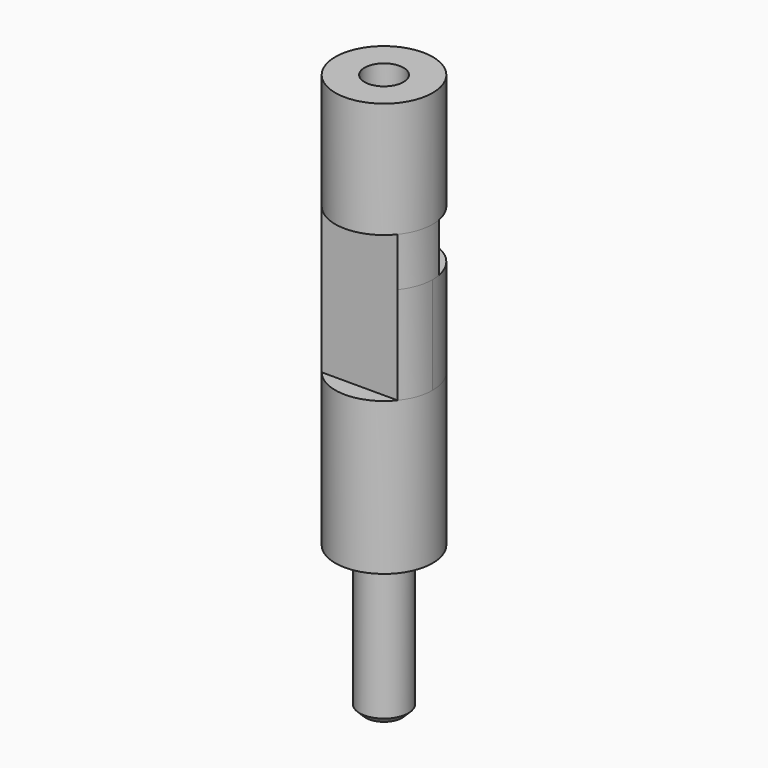
from build123d import *
from build123d import SkipClean  # not in build123d's __all__

# Parameters (mm, degrees)
F2_SIZE   = 0.5
F4_DEPTH  = 8
F6_DEPTH  = 4
F7_R      = 4
F8_DEPTH  = 9.5
F10_D     = 3.2
F10_DEPTH = 14
F10_TIP   = 0.9613769904
F11_R     = 1.6
F12_DEPTH = 2.53


# Not quite as in the source:
# - after a boolean that leaves OpenCascade's solid faulty, fix() repairs it


with BuildPart() as f1:
    # F0 (on Front) → F1 (revolve)
    with BuildSketch(Plane.XZ):
        Polygon((-2, 0), (0, 0), (0, 24.5), (-4, 24.5), (-4, 12), (-2, 12), align=None)
    revolve(axis=Axis((0, 0, 12.25), (0, 0, -1)))

    # F2
    f2_edges = [f1.edges().sort_by_distance(p)[0] for p in [
        (2, 0, 0),
    ]]
    chamfer(f2_edges, length=F2_SIZE)

    # F3 (on face) → F4 (join)
    with BuildSketch(Plane.XY.offset(24.5)):
        with BuildLine():
            Line((-3.1224989992, -2.5), (3.1224989992, -2.5))
            ThreePointArc((3.1224989992, -2.5), (3.7742546282, -1.3247648854), (4, 0))
            ThreePointArc((4, 0), (-1.3247648854, 3.7742546282), (-3.1224989992, -2.5))
        make_face()
    with SkipClean():  # cleaning this boolean's faces spoils the solid; the shape is the same uncleaned
        extrude(amount=F4_DEPTH)

    # F5 (on face) → F6 (join)
    with BuildSketch(Plane.XY.offset(32.5)):
        with BuildLine():
            Line((-3.1224989992, -2.5), (3.1224989992, -2.5))
            ThreePointArc((3.1224989992, -2.5), (3.8760324942, -0.9881154306), (3.9382737335, 0.7))
            Line((3.9382737335, 0.7), (2.1, 2.5))
            Line((2.1, 2.5), (-2.1, 2.5))
            Line((-2.1, 2.5), (-3.7080992435, 1.5))
            ThreePointArc((-3.7080992435, 1.5), (-3.9578110223, -0.5794237754), (-3.1224989992, -2.5))
        make_face()
    extrude(amount=F6_DEPTH)

    add(f1.part.fix(), mode=Mode.REPLACE)

    # F7 (on face) → F8 (join)
    with BuildSketch(Plane.XY.offset(36.5)):
        Circle(F7_R)
    extrude(amount=F8_DEPTH)

    # F10
    with Locations(Plane.XY.offset(46)):
        with Locations((0, 0)):
            Hole(F10_D / 2, depth=F10_DEPTH)
            with Locations((0, 0, -(F10_DEPTH + F10_TIP / 2))):  # 118° drill point
                Cone(0, F10_D / 2, F10_TIP, mode=Mode.SUBTRACT)

    # F11 (on face) → F12 (cut)
    with BuildSketch(Plane(origin=(0, 2.5, 0), x_dir=(-1, 0, 0), z_dir=(0, 1, 0))):
        with Locations((0, 34.5)):
            Circle(F11_R)
    extrude(amount=-F12_DEPTH, mode=Mode.SUBTRACT)


solid = f1.part
